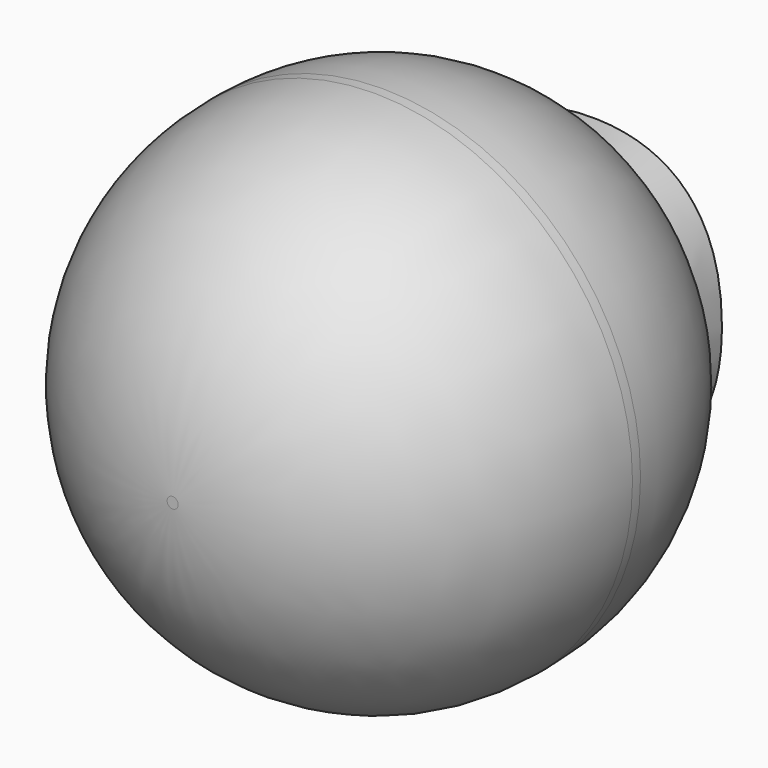
from build123d import *

# Parameters (mm, degrees)
F0_R         = 25.4508928741
F0_TEXT_SIZE = 38.9611361445
F1_DEPTH     = 50.8
F2_R         = 24.9057030892
F3_TEXT_SIZE = 37.9809812229
F4_DEPTH     = 12.7


# Not quite as in the source:
# - Text() gives the source's letters only with a copy of the font that has no kerning and outlines rounded to 1/6400 em; it was checked with that copy


with BuildPart() as f1:
    # F0 (on Front) → F1 (new body)
    with BuildSketch(Plane.XZ):
        with Locations((-26.2877400964, 24.25882034)):
            Circle(F0_R)
        with BuildLine():
            add(Edge.make_bspline(
                [(-16.1114416284, 34.7053328156), (-12.7145175708, 31.0131563981), (-12.7145175708, 24.091467055)],
                knots=[0, 0, 0, 1, 1, 1], degree=2))
            add(Edge.make_bspline(
                [(-12.7145175708, 24.091467055), (-12.7145175708, 17.1819530668), (-16.1388361773, 13.4715136168)],
                knots=[0, 0, 0, 1, 1, 1], degree=2))
            add(Edge.make_bspline(
                [(-16.1388361773, 13.4715136168), (-19.5631547837, 9.7610741668), (-25.9552161824, 9.7610741668)],
                knots=[0, 0, 0, 1, 1, 1], degree=2))
            add(Edge.make_bspline(
                [(-25.9552161824, 9.7610741668), (-32.3472775811, 9.7610741668), (-35.7715961876, 13.4715136168)],
                knots=[0, 0, 0, 1, 1, 1], degree=2))
            add(Edge.make_bspline(
                [(-35.7715961876, 13.4715136168), (-39.195914794, 17.1819530668), (-39.195914794, 24.1279931201)],
                knots=[0, 0, 0, 1, 1, 1], degree=2))
            add(Edge.make_bspline(
                [(-39.195914794, 24.1279931201), (-39.195914794, 31.0740331734), (-35.7624646713, 34.7357712032)],
                knots=[0, 0, 0, 1, 1, 1], degree=2))
            add(Edge.make_bspline(
                [(-35.7624646713, 34.7357712032), (-32.3290145485, 38.397509233), (-25.9186901173, 38.397509233)],
                knots=[0, 0, 0, 1, 1, 1], degree=2))
            add(Edge.make_bspline(
                [(-25.9186901173, 38.397509233), (-19.508365686, 38.397509233), (-16.1114416284, 34.7053328156)],
                knots=[0, 0, 0, 1, 1, 1], degree=2))
        make_face(mode=Mode.SUBTRACT)
        with Locations((-41.4605308324, 10.1445978507)):
            Text('O', F0_TEXT_SIZE, font='Open Sans', font_style=FontStyle.BOLD, text_align=(TextAlign.LEFT, TextAlign.BOTTOM))
        with BuildLine():
            add(Edge.make_bspline(
                [(-31.2241010782, 31.116646916), (-33.0108344311, 28.7485403597), (-33.0108344311, 24.091467055)],
                knots=[0, 0, 0, 1, 1, 1], degree=2))
            add(Edge.make_bspline(
                [(-33.0108344311, 24.091467055), (-33.0108344311, 19.4283060727), (-31.2423641108, 17.0693310327)],
                knots=[0, 0, 0, 1, 1, 1], degree=2))
            add(Edge.make_bspline(
                [(-31.2423641108, 17.0693310327), (-29.4738937905, 14.7103559927), (-25.9552161824, 14.7103559927)],
                knots=[0, 0, 0, 1, 1, 1], degree=2))
            add(Edge.make_bspline(
                [(-25.9552161824, 14.7103559927), (-18.8995979337, 14.7103559927), (-18.8995979337, 24.091467055)],
                knots=[0, 0, 0, 1, 1, 1], degree=2))
            add(Edge.make_bspline(
                [(-18.8995979337, 24.091467055), (-18.8995979337, 33.4847534723), (-25.9186901173, 33.4847534723)],
                knots=[0, 0, 0, 1, 1, 1], degree=2))
            add(Edge.make_bspline(
                [(-25.9186901173, 33.4847534723), (-29.4373677253, 33.4847534723), (-31.2241010782, 31.116646916)],
                knots=[0, 0, 0, 1, 1, 1], degree=2))
        make_face()
    extrude(amount=F1_DEPTH)

    # F2
    f2_edges = [f1.edges().sort_by_distance(p)[0] for p in [
        (-51.738633, 0, 24.25882),
        (-51.738633, -50.8, 24.25882),
    ]]
    fillet(f2_edges, radius=F2_R)

    # F3 (on Front) → F4 (join)
    with BuildSketch(Plane.XZ):
        with Locations((-40.7548230141, 9.791742079)):
            Text('O', F3_TEXT_SIZE, font='Open Sans', font_style=FontStyle.BOLD, text_align=(TextAlign.LEFT, TextAlign.BOTTOM))
    extrude(amount=F4_DEPTH)


solid = f1.part
